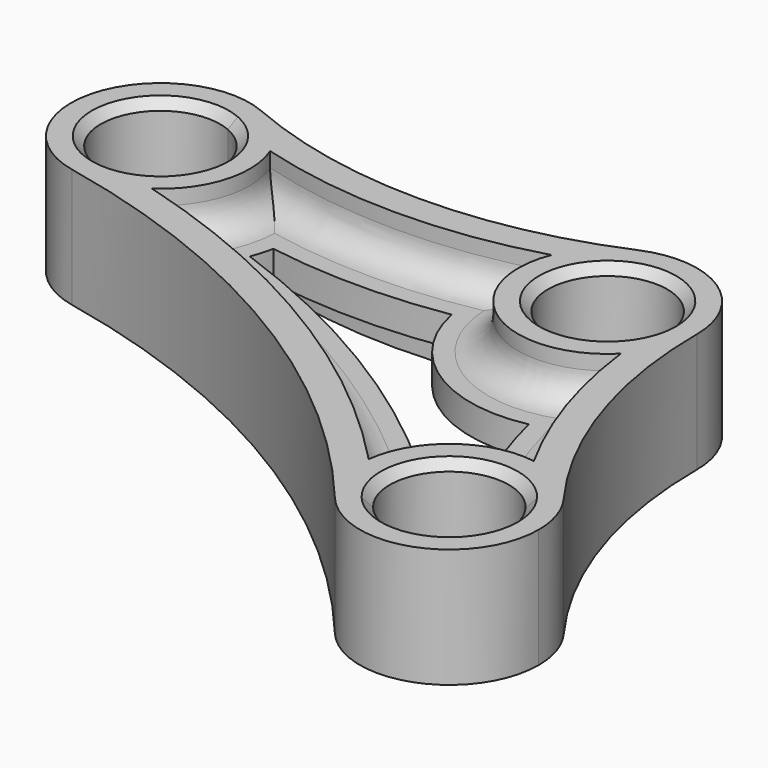
from build123d import *

# Parameters (mm, degrees)
F1_DEPTH = 10
F2_DEPTH = 2.5
F3_R     = 5
F5_DEPTH = 12.501
F6_SIZE  = 1.5


# Not quite as in the source:
# - ends of sketch curves that miss each other by under 0.0002 mm in the source are joined


with BuildPart() as f1:
    # F0 (on Top) → F1 (new body, symmetric)
    with BuildSketch(Plane.XY):
        with BuildLine():
            ThreePointArc((-61.1270550584, 5.6233035221), (-64.3120758187, 10.4909176924), (-69.1094465162, 13.7807899309))
            ThreePointArc((-69.1094465162, 13.7807899309), (-89.3390658482, 4.5099582499), (-78.083775001, -14.6865061725))
            ThreePointArc((-78.083775001, -14.6865061725), (-72.0748340452, -14.7053930071), (-66.5406341793, -12.3643761411))
            ThreePointArc((-66.5406341793, -12.3643761411), (-71.7812655501, -10.9856736162), (-77.0668876123, -9.7910032715))
            ThreePointArc((-77.0668876123, -9.7910032715), (-84.570415019, 3.0066388333), (-71.0840021309, 9.1871932872))
            ThreePointArc((-71.0840021309, 9.1871932872), (-66.1610088951, 7.2502451775), (-61.1270550584, 5.6233035221))
        make_face()
        with BuildLine():
            ThreePointArc((-60.0331133604, 0), (-60.3091384465, 2.8643607899), (-61.1270550584, 5.6233035221))
            ThreePointArc((-61.1270550584, 5.6233035221), (-66.1610088951, 7.2502451775), (-71.0840021309, 9.1871932872))
            ThreePointArc((-71.0840021309, 9.1871932872), (-66.6817328669, 5.5004039718), (-65.0331133604, 0))
            ThreePointArc((-65.0331133604, 0), (-68.7219226752, -7.7568596826), (-77.0668877875, -9.791004115))
            ThreePointArc((-77.0668877875, -9.791004115), (-71.7812655501, -10.9856736162), (-66.5406341793, -12.3643761411))
            ThreePointArc((-66.5406341793, -12.3643761411), (-61.7593198612, -6.9861581818), (-60.0331133604, 0))
        make_face()
        with BuildLine():
            ThreePointArc((-13.906058302, 5.6233035221), (-8.2506059576, -12.5270707403), (10.6578947368, -10.5550594398))
            ThreePointArc((10.6578947368, -10.5550594398), (10.1646331199, -5.2877713941), (10, 0))
            ThreePointArc((10, 0), (-5.5004039718, -8.3513804935), (-3.9491112295, 9.1871932872))
            ThreePointArc((-3.9491112295, 9.1871932872), (-8.8721044653, 7.2502451775), (-13.906058302, 5.6233035221))
        make_face()
        with BuildLine():
            ThreePointArc((10.6578947368, -10.5550594398), (13.8720658348, -5.7066443269), (15, 0))
            ThreePointArc((15, 0), (8.2506059576, 12.5270707403), (-5.9236668442, 13.7807899309))
            ThreePointArc((-5.9236668442, 13.7807899309), (-10.7210375417, 10.4909176924), (-13.906058302, 5.6233035221))
            ThreePointArc((-13.906058302, 5.6233035221), (-8.8721044653, 7.2502451775), (-3.9491112295, 9.1871932872))
            ThreePointArc((-3.9491112295, 9.1871932872), (5.5004039718, 8.3513804935), (10, 0))
            ThreePointArc((10, 0), (10.1646331199, -5.2877713941), (10.6578947368, -10.5550594398))
        make_face()
        with BuildLine():
            ThreePointArc((26.5285242746, -50.3652361455), (23.527969189, -46.0081385383), (20.8042767721, -41.4728182632))
            ThreePointArc((20.8042767721, -41.4728182632), (9.3957138654, -44.3489563966), (3.5718338704, -54.5719647583))
            ThreePointArc((3.5718338704, -54.5719647583), (7.2428277606, -58.5580457504), (10.7722421784, -62.6700126379))
            ThreePointArc((10.7722421784, -62.6700126379), (12.3181130698, -48.4091450465), (26.5285242746, -50.3652361455))
        make_face()
        with BuildLine():
            ThreePointArc((33.4730565422, -56.2905580449), (32.7252146942, -51.6133806899), (30.5562581408, -47.4025751957))
            ThreePointArc((30.5562581408, -47.4025751957), (26.2662839534, -43.4739435732), (20.8042767721, -41.4728182632))
            ThreePointArc((20.8042767721, -41.4728182632), (23.527969189, -46.0081385383), (26.5285242746, -50.3652361455))
            ThreePointArc((26.5285242746, -50.3652361455), (27.9744953102, -53.1724398082), (28.4730565422, -56.2905580449))
            ThreePointArc((28.4730565422, -56.2905580449), (21.8636206345, -65.6982184946), (10.772241515, -62.6700131875))
            ThreePointArc((10.772241515, -62.6700131875), (7.2428277606, -58.5580457504), (3.5718338704, -54.5719647583))
            ThreePointArc((3.5718338704, -54.5719647583), (4.0929857429, -60.5582932532), (6.9218340013, -65.8597407588))
            ThreePointArc((6.9218340013, -65.8597407588), (23.5589026806, -70.4020487194), (33.4730565422, -56.2905580449))
        make_face()
        with BuildLine():
            ThreePointArc((-66.5406341793, -12.3643761411), (-72.0748340452, -14.7053930071), (-78.083775001, -14.6865061725))
            ThreePointArc((-78.083775001, -14.6865061725), (-31.2272831079, -33.0410645358), (6.9218340013, -65.8597407588))
            ThreePointArc((6.9218340013, -65.8597407588), (4.0929857429, -60.5582932532), (3.5718338704, -54.5719647583))
            ThreePointArc((3.5718338704, -54.5719647583), (-28.6485123869, -28.7573803523), (-66.5406341793, -12.3643761411))
        make_face()
        with BuildLine():
            ThreePointArc((-13.906058302, 5.6233035221), (-10.7210375417, 10.4909176924), (-5.9236668442, 13.7807899309))
            ThreePointArc((-5.9236668442, 13.7807899309), (-37.5165566802, 7.2783362288), (-69.1094465162, 13.7807899309))
            ThreePointArc((-69.1094465162, 13.7807899309), (-64.3120758187, 10.4909176924), (-61.1270550584, 5.6233035221))
            ThreePointArc((-61.1270550584, 5.6233035221), (-37.5165566802, 2.2783362288), (-13.906058302, 5.6233035221))
        make_face()
        with BuildLine():
            ThreePointArc((30.5562581408, -47.4025751957), (18.988489856, -24.9449458936), (15, 0))
            ThreePointArc((15, 0), (13.8720658348, -5.7066443269), (10.6578947368, -10.5550594398))
            ThreePointArc((10.6578947368, -10.5550594398), (14.237770472, -26.5040050119), (20.8042767721, -41.4728182632))
            ThreePointArc((20.8042767721, -41.4728182632), (26.2662839534, -43.4739435732), (30.5562581408, -47.4025751957))
        make_face()
    extrude(amount=F1_DEPTH, both=True)

    # F0 (on Top) → F2 (join, symmetric)
    with BuildSketch(Plane.XY):
        with BuildLine():
            ThreePointArc((20.8042767721, -41.4728182632), (14.237770472, -26.5040050119), (10.6578947368, -10.5550594398))
            ThreePointArc((10.6578947368, -10.5550594398), (-8.2506059576, -12.5270707403), (-13.906058302, 5.6233035221))
            ThreePointArc((-13.906058302, 5.6233035221), (-37.5165566802, 2.2783362288), (-61.1270550584, 5.6233035221))
            ThreePointArc((-61.1270550584, 5.6233035221), (-60.3091384465, 2.8643607899), (-60.0331133604, 0))
            ThreePointArc((-60.0331133604, 0), (-61.7593198612, -6.9861581818), (-66.5406341793, -12.3643761411))
            ThreePointArc((-66.5406341793, -12.3643761411), (-28.6485123869, -28.7573803523), (3.5718338704, -54.5719647583))
            ThreePointArc((3.5718338704, -54.5719647583), (9.3957138654, -44.3489563966), (20.8042767721, -41.4728182632))
        make_face()
    extrude(amount=F2_DEPTH, both=True)

    # F3
    f3_edges = [f1.edges().sort_by_distance(p)[0] for p in [
        (14.23777, -26.504005, 2.5),
        (-8.250606, -12.527071, 2.5),
        (-37.516557, 2.278336, 2.5),
        (-60.669521, -4.322872, 2.5),
        (-28.648512, -28.75738, 2.5),
        (9.395714, -44.348956, 2.5),
        (14.23777, -26.504005, -2.5),
        (-8.250606, -12.527071, -2.5),
        (-37.516557, 2.278336, -2.5),
        (-60.669521, -4.322872, -2.5),
        (-28.648512, -28.75738, -2.5),
        (9.395714, -44.348956, -2.5),
    ]]
    fillet(f3_edges, radius=F3_R)

    # F4 (on face) → F5 (cut, through all)
    with BuildSketch(Plane.XY.offset(2.5)):
        with BuildLine():
            ThreePointArc((4.7631578947, -22.5013849989), (-12.650929135, -19.2081751351), (-22.5534813546, -4.5100419942))
            ThreePointArc((-22.5534813546, -4.5100419942), (-37.5165566802, -5.7216637712), (-52.4796320058, -4.5100419942))
            ThreePointArc((-52.4796320058, -4.5100419942), (-52.9254779245, -6.3444822825), (-53.5202661907, -8.1361788731))
            ThreePointArc((-53.5202661907, -8.1361788731), (-24.5224799443, -21.9034868397), (1.2149484666, -41.0866866415))
            ThreePointArc((1.2149484666, -41.0866866415), (4.7912073526, -37.8025348204), (8.9772080845, -35.3423155872))
            ThreePointArc((8.9772080845, -35.3423155872), (6.6366194576, -28.9984996013), (4.7631578947, -22.5013849989))
        make_face()
    extrude(amount=-F5_DEPTH, mode=Mode.SUBTRACT)

    # F6
    f6_edges = [f1.edges().sort_by_distance(p)[0] for p in [
        (-84.570415, 3.006639, 10),
        (3.949111, -9.187193, 10),
        (12.318113, -48.409145, 10),
    ]]
    chamfer(f6_edges, length=F6_SIZE)


solid = f1.part
